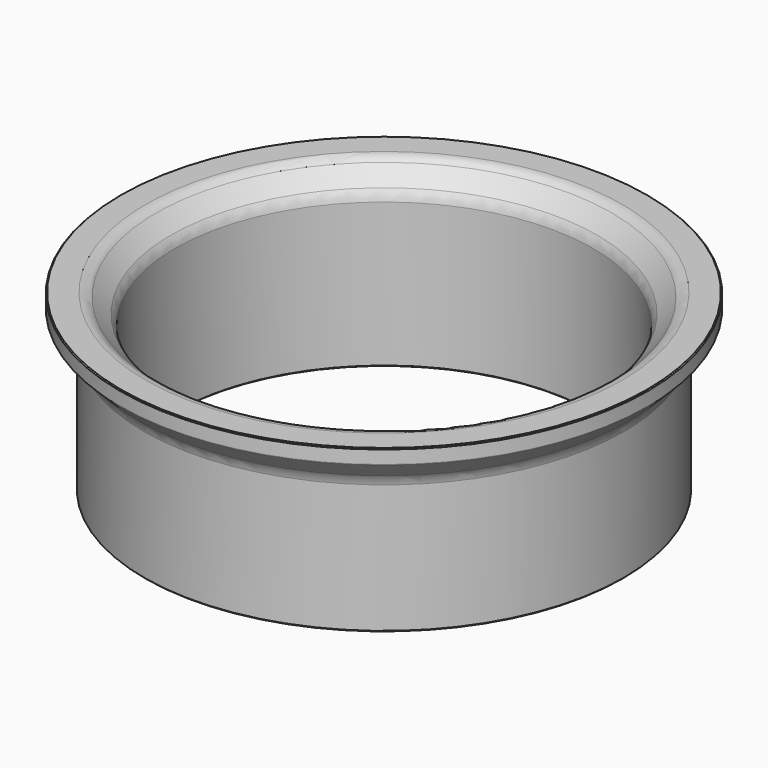
from build123d import *

# Parameters (mm, degrees)
F2_R = 1.5
F3_R = 1.5
F4_R = 1.5


# Not quite as in the source:
# - a fillet or chamfer that OpenCascade refuses, or shapes differently, is made with other operations: its cross-section is extruded or revolved along the edge and cut away or added


with BuildPart() as f1:
    # F0 (on Front) → F1 (revolve)
    with BuildSketch(Plane.XZ):
        Polygon((21.6, 15.6), (21.6, 0), (24.8, 0), (24.8, 14), (27.3, 16.5), (27.3, 18), (24, 18), align=None)
    revolve(axis=Axis((0, 0, 6.0077635571), (0, 0, -1)))

    # F2
    f2_edges = [f1.edges().sort_by_distance(p)[0] for p in [
        (-21.6, 0, 15.6),
    ]]
    fillet(f2_edges, radius=F2_R)

    # F3
    f3_edges = [f1.edges().sort_by_distance(p)[0] for p in [
        (-24, 0, 18),
    ]]
    fillet(f3_edges, radius=F3_R)

    # F4
    f4_edges = [f1.edges().sort_by_distance(p)[0] for p in [
        (-24.8, 0, 14),
    ]]
    fillet(f4_edges, radius=F4_R)

    # F5: chamfer of 0.1 on 5 edges, made by hand

    # F5_s1 → F5_t2 (revolve, cut)
    with BuildSketch(Plane.XZ):
        Polygon((27.3, 17.9), (27.2, 18), (27.3, 18), align=None)
    revolve(axis=Axis((0, 0, 18), (0, 0, -1)), mode=Mode.SUBTRACT)

    # F5_s3 → F5_t4 (revolve, cut)
    with BuildSketch(Plane.XZ):
        Polygon((27.2707106781, 16.4707106781), (27.3, 16.5414213562), (27.3, 16.5), align=None)
    revolve(axis=Axis((0, 0, 16.5), (0, 0, -1)), mode=Mode.SUBTRACT)

    # F5_s5 → F5_t6 (revolve, cut)
    with BuildSketch(Plane.XZ):
        Polygon((24.8, 0.1), (24.7, 0), (24.8, 0), align=None)
    revolve(axis=Axis((0, 0, 0), (0, 0, -1)), mode=Mode.SUBTRACT)

    # F5_s7 → F5_t8 (revolve, cut)
    with BuildSketch(Plane.XZ):
        Polygon((21.7, 0), (21.6, 0.1), (21.6, 0), align=None)
    revolve(axis=Axis((0, 0, 0), (0, 0, -1)), mode=Mode.SUBTRACT)


solid = f1.part
